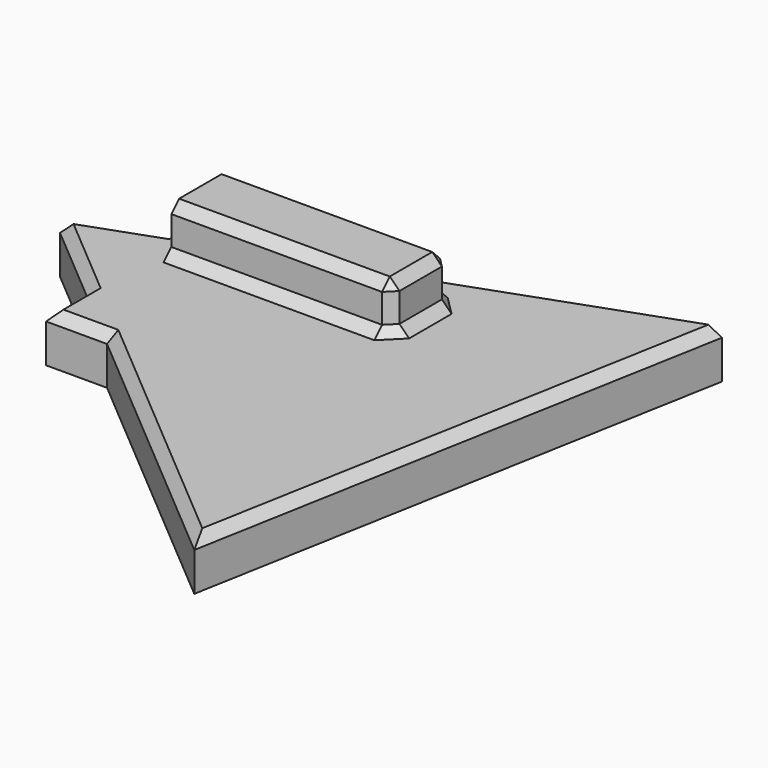
from build123d import *

# Parameters (mm, degrees)
F0_W     = 127
F0_H     = 38.1
F1_DEPTH = 25.4
F2_W     = 115.9340298213
F2_H     = 38.1
F3_DEPTH = 25.4
F4_W     = 127
F4_H     = 68.654977391
F5_DEPTH = 25.4
F7_DEPTH = 25.4
F8_SIZE  = 5.08


# Not quite as in the source:
# - the program builds the solid bodies; features that only make, move or delete a surface that nothing else refers to are left out


with BuildPart() as f1:
    # F0 (on Top) → F1 (new body)
    with BuildSketch(Plane.XY):
        with Locations((3.9197548818, 19.05)):
            Rectangle(F0_W, F0_H)
    extrude(amount=F1_DEPTH)

    # F2 (on face) → F3 (join)
    with BuildSketch(Plane.XY.offset(25.4)):
        with Locations((9.4527399712, 19.05)):
            Rectangle(F2_W, F2_H)
    extrude(amount=F3_DEPTH)

    # F4 (on Top) → F5 (join)
    with BuildSketch(Plane.XY):
        with Locations((3.9833925518, -34.3274886955)):
            Rectangle(F4_W, F4_H)
    extrude(amount=F5_DEPTH)

    # F6 (on Top) → F7 (join)
    with BuildSketch(Plane.XY):
        Polygon((115.0657710181, -189.4061209801), (166.3690629853, 93.5014354232), (-104.2877137661, -3.5223886371), align=None)
    extrude(amount=F7_DEPTH)

    # F8
    f8_edges = [f1.edges().sort_by_distance(p)[0] for p in [
        (140.717417, -47.952343, 25.4),
        (43.819127, -129.030549, 25.4),
        (-43.472062, -68.654977, 25.4),
        (-59.516607, -55.058567, 25.4),
        (-81.902161, -22.492273, 25.4),
        (9.45274, 0, 50.8),
        (-23.879261, 38.1, 0),
        (9.45274, 38.1, 50.8),
        (67.419755, 19.05, 50.8),
        (67.419755, 0, 38.1),
        (67.419755, 19.05, 25.4),
        (67.419755, 38.1, 38.1),
        (39.620739, 38.1, 25.4),
        (9.45274, 0, 25.4),
    ]]
    chamfer(f8_edges, length=F8_SIZE)


solid = f1.part
